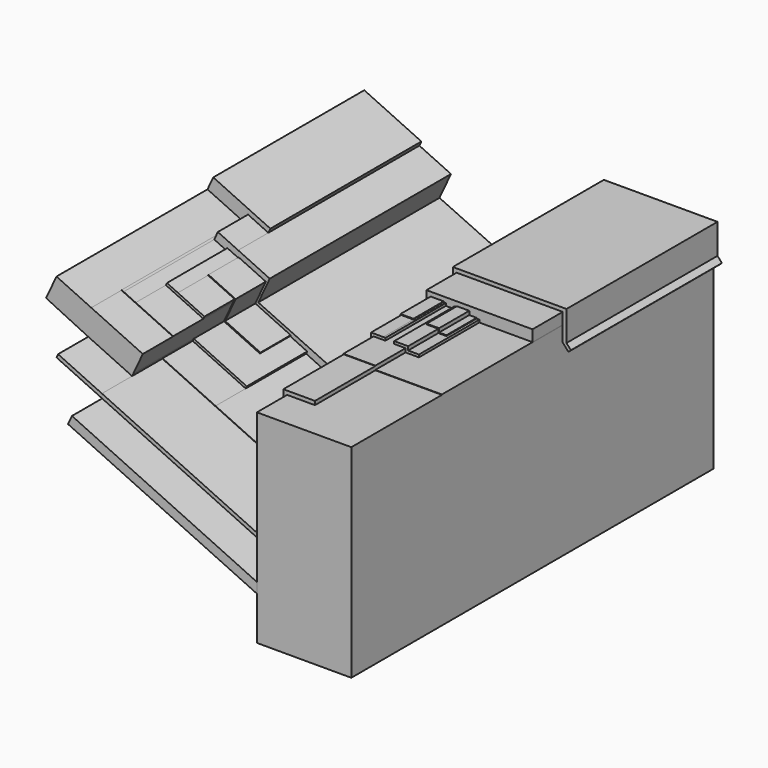
from build123d import *

# Parameters (mm, degrees)
F1_DEPTH  = 120
F2_DEPTH  = 120
F3_DEPTH  = 110
F4_DEPTH  = 100
F5_DEPTH  = 100
F6_DEPTH  = 90
F7_DEPTH  = 90
F8_DEPTH  = 90
F9_DEPTH  = 80
F10_DEPTH = 80
F11_DEPTH = 80
F12_DEPTH = 80
F13_DEPTH = 80
F14_DEPTH = 70
F15_DEPTH = 70
F16_DEPTH = 70
F17_DEPTH = 70
F18_DEPTH = 60
F19_DEPTH = 50
F20_DEPTH = 50


with BuildPart() as f1:
    # F0 (on Front) → F1 (new body)
    with BuildSketch(Plane.XZ):
        Polygon((45.1297726456, 37.9975503451), (37.7532724798, 37.9975503451), (37.7532724798, -1.5682141957), (37.7532724798, -4.3017355894), (37.7532724798, -15.7766969041), (62.7532724798, -15.7766969041), (62.7532724798, 33.9434424275), (62.7532724798, 37.9975503451), align=None)
    extrude(amount=F1_DEPTH)


with BuildPart() as f2:
    # F0 (on Front) → F2 (new body)
    with BuildSketch(Plane.XZ):
        Polygon((37.7532724798, -4.3017355894), (37.7532724798, -1.5682141957), (-11.241981874, 21.2279597303), (-12.2874860827, 18.9808833218), align=None)
    extrude(amount=F2_DEPTH)


with BuildPart() as f3:
    # F0 (on Front) → F3 (new body)
    with BuildSketch(Plane.XZ):
        Polygon((37.7532724798, -1.5682141957), (37.7532724798, 37.9975503451), (45.1297726456, 37.9975503451), (45.1297726456, 38.0975503451), (45.1297726456, 38.9975503451), (36.7532724798, 38.9975503451), (36.7532724798, 9.1857140463), (36.7532724798, 0), (27.1622682206, 4.4624362931), (-11.3030609789, 22.3593192896), (-22.921301212, 27.7649739506), (-23.3431488548, 26.8583072168), (-11.241981874, 21.2279597303), align=None)
    extrude(amount=F3_DEPTH)


with BuildPart() as f4:
    # F0 (on Front) → F4 (new body)
    with BuildSketch(Plane.XZ):
        Polygon((-34.093962769, 33.1498159787), (-22.921301212, 27.7649739506), (-11.3030609789, 22.3593192896), (-11.2608762147, 22.449985963), (-10.978238294, 23.0574526746), (-8.4765384307, 28.4342944867), (-22.1272858391, 34.785620064), (-31.3387730508, 39.0714772835), align=None)
    extrude(amount=F4_DEPTH)


with BuildPart() as f5:
    # F0 (on Front) → F5 (new body)
    with BuildSketch(Plane.XZ):
        Polygon((36.7532724798, 0), (36.7532724798, 9.1857140463), (27.1622682206, 4.4624362931), align=None)
    extrude(amount=F5_DEPTH)


with BuildPart() as f6:
    # F0 (on Front) → F6 (new body)
    with BuildSketch(Plane.XZ):
        Polygon((-22.0851010748, 34.8762867374), (-22.1272858391, 34.785620064), (-8.4765384307, 28.4342944867), (-8.4343536664, 28.5249611601), (-18.3601163214, 33.1431515301), (-21.5557715405, 34.6300039435), align=None)
    extrude(amount=F6_DEPTH)


with BuildPart() as f7:
    # F0 (on Front) → F7 (new body)
    with BuildSketch(Plane.XZ):
        Polygon((36.7532724798, 38.9975503451), (45.1297726456, 38.9975503451), (45.1297726456, 39.0975503451), (42.1224348247, 39.0975503451), (39.793651551, 39.0975503451), (36.6532724798, 39.0975503451), (36.6532724798, 36.1267757076), (36.6532724798, 15.0731514328), (36.6532724798, 9.247935752), (27.1610418439, 4.5733010027), (20.5657351542, 7.641919798), (2.7888639592, 15.9130197845), (-11.2608762147, 22.449985963), (-11.3030609789, 22.3593192896), (27.1622682206, 4.4624362931), (36.7532724798, 9.1857140463), align=None)
    extrude(amount=F7_DEPTH)


with BuildPart() as f8:
    # F0 (on Front) → F8 (new body)
    with BuildSketch(Plane.XZ):
        Polygon((45.1297726456, 38.0975503451), (45.1297726456, 37.9975503451), (62.7532724798, 37.9975503451), (62.7532724798, 38.0975503451), (48.6693568528, 38.0975503451), align=None)
    extrude(amount=F8_DEPTH)


with BuildPart() as f9:
    # F0 (on Front) → F9 (new body)
    with BuildSketch(Plane.XZ):
        Polygon((-18.3601163214, 33.1431515301), (-8.4343536664, 28.5249611601), (-8.1517157457, 29.1324278718), (-15.1795170811, 32.4022747921), (-18.0774784007, 33.7506182417), align=None)
    extrude(amount=F9_DEPTH)


with BuildPart() as f10:
    # F0 (on Front) → F10 (new body)
    with BuildSketch(Plane.XZ):
        Polygon((-10.978238294, 23.0574526746), (-11.2608762147, 22.449985963), (2.7888639592, 15.9130197845), (3.0715018799, 16.5204864961), (-1.4491225171, 18.6238114276), align=None)
    extrude(amount=F10_DEPTH)


with BuildPart() as f11:
    # F0 (on Front) → F11 (new body)
    with BuildSketch(Plane.XZ):
        Polygon((20.987582797, 8.5485865319), (20.5657351542, 7.641919798), (27.1610418439, 4.5733010027), (36.6532724798, 9.247935752), (36.6532724798, 15.0731514328), (35.6532724798, 15.0731514328), (35.6532724798, 13.1126534771), (35.6532724798, 9.8701528088), (27.1487780767, 5.6819480984), (22.5392122095, 7.8266551036), (22.3868255866, 7.8975565001), align=None)
    extrude(amount=F11_DEPTH)


with BuildPart() as f12:
    # F0 (on Front) → F12 (new body)
    with BuildSketch(Plane.XZ):
        Polygon((36.6532724798, 39.0975503451), (39.793651551, 39.0975503451), (39.793651551, 39.7675503451), (39.2196215689, 39.7700648543), (35.9832724798, 39.7842415175), (35.9832724798, 36.6213790533), (35.9832724798, 36.1267757076), (36.6532724798, 36.1267757076), align=None)
    extrude(amount=F12_DEPTH)


with BuildPart() as f13:
    # F0 (on Front) → F13 (new body)
    with BuildSketch(Plane.XZ):
        Polygon((45.1297726456, 38.9975503451), (45.1297726456, 38.0975503451), (48.6693568528, 38.0975503451), (48.6693568528, 38.7675503451), (47.9532927275, 38.7675503451), (45.7997726456, 38.7675503451), (45.7997726456, 39.7675503451), (42.7247062325, 39.7675503451), (42.1224348247, 39.7675503451), (42.1224348247, 39.0975503451), (45.1297726456, 39.0975503451), align=None)
    extrude(amount=F13_DEPTH)


with BuildPart() as f14:
    # F0 (on Front) → F14 (new body)
    with BuildSketch(Plane.XZ):
        Polygon((-8.4765384307, 28.4342944867), (-10.978238294, 23.0574526746), (-1.4491225171, 18.6238114276), (-1.3221520646, 18.8967058894), (-10.6699344948, 23.2459776078), (-7.8860128704, 29.22939169), (-15.0951475526, 32.5836081388), (-15.1795170811, 32.4022747921), (-8.1517157457, 29.1324278718), (-8.4343536664, 28.5249611601), align=None)
    extrude(amount=F14_DEPTH)


with BuildPart() as f15:
    # F0 (on Front) → F15 (new body)
    with BuildSketch(Plane.XZ):
        Polygon((35.6532724798, 9.8701528088), (35.6532724798, 13.1126534771), (35.4532724798, 13.1126534771), (35.4532724798, 9.9945962202), (27.1500502265, 5.9019444203), (22.623581738, 8.0079884503), (22.5392122095, 7.8266551036), (27.1487780767, 5.6819480984), align=None)
    extrude(amount=F15_DEPTH)


with BuildPart() as f16:
    # F0 (on Front) → F16 (new body)
    with BuildSketch(Plane.XZ):
        Polygon((35.9832724798, 39.7842415175), (39.2196215689, 39.7700648543), (39.2196215689, 39.9700648543), (35.7832724798, 39.9700648543), (35.7832724798, 36.6213790533), (35.9832724798, 36.6213790533), align=None)
    extrude(amount=F16_DEPTH)


with BuildPart() as f17:
    # F0 (on Front) → F17 (new body)
    with BuildSketch(Plane.XZ):
        Polygon((45.7997726456, 38.7675503451), (47.9532927275, 38.7675503451), (47.9532927275, 38.9675503451), (45.9997726456, 38.9675503451), (45.9997726456, 39.9675503451), (42.7247062325, 39.9675503451), (42.7247062325, 39.7675503451), (45.7997726456, 39.7675503451), align=None)
    extrude(amount=F17_DEPTH)


with BuildPart() as f18:
    # F0 (on Front) → F18 (new body)
    with BuildSketch(Plane.XZ):
        Polygon((48.6693568528, 38.0975503451), (62.7532724798, 38.0975503451), (62.7532724798, 41.0975503451), (47.1063793285, 41.0975503451), (46.2950781567, 41.0975503451), (34.6532724798, 41.0975503451), (34.6532724798, 33.1212431192), (34.6532724798, 16.1968208849), (33.6532724798, 13.4902799919), (33.6532724798, 11.3371306488), (27.2846735988, 8.1965293972), (23.4195049672, 9.6229607519), (20.8119284671, 9.6229607519), (-9.8889558036, 23.7389743125), (-6.8439622262, 30.2835039038), (-15.2163269439, 34.1789399985), (-20.6001537113, 36.6838897736), (-21.5557715405, 34.6300039435), (-18.3601163214, 33.1431515301), (-18.0774784007, 33.7506182417), (-15.1795170811, 32.4022747921), (-15.0951475526, 32.5836081388), (-7.8860128704, 29.22939169), (-10.6699344948, 23.2459776078), (-1.3221520646, 18.8967058894), (-1.4491225171, 18.6238114276), (3.0715018799, 16.5204864961), (2.7888639592, 15.9130197845), (20.5657351542, 7.641919798), (20.987582797, 8.5485865319), (22.3868255866, 7.8975565001), (22.5392122095, 7.8266551036), (22.623581738, 8.0079884503), (27.1500502265, 5.9019444203), (35.4532724798, 9.9945962202), (35.4532724798, 13.1126534771), (35.6532724798, 13.1126534771), (35.6532724798, 15.0731514328), (36.6532724798, 15.0731514328), (36.6532724798, 36.1267757076), (35.9832724798, 36.1267757076), (35.9832724798, 36.6213790533), (35.7832724798, 36.6213790533), (35.7832724798, 39.9700648543), (39.2196215689, 39.9700648543), (39.2196215689, 39.7700648543), (39.793651551, 39.7675503451), (39.793651551, 39.0975503451), (42.1224348247, 39.0975503451), (42.1224348247, 39.7675503451), (42.7247062325, 39.7675503451), (42.7247062325, 39.9675503451), (45.9997726456, 39.9675503451), (45.9997726456, 38.9675503451), (47.9532927275, 38.9675503451), (47.9532927275, 38.7675503451), (48.6693568528, 38.7675503451), align=None)
    extrude(amount=F18_DEPTH)


with BuildPart() as f19:
    # F0 (on Front) → F19 (new body)
    with BuildSketch(Plane.XZ):
        Polygon((62.7532724798, 38.0975503451), (62.7532724798, 37.9975503451), (62.7532724798, 33.9434424275), (64.2652862209, 32.2634628909), (64.9253694473, 32.85755043), (63.7534983963, 34.1596016824), (63.7534983963, 42.0975503451), (33.6532724798, 42.0975503451), (33.6532724798, 33.7673542435), (32.3305874402, 33.1794772946), (32.7367356742, 32.2656700874), (34.6532724798, 33.1212431192), (34.6532724798, 41.0975503451), (46.2950781567, 41.0975503451), (47.1063793285, 41.0975503451), (62.7532724798, 41.0975503451), align=None)
    extrude(amount=F19_DEPTH)


with BuildPart() as f20:
    # F0 (on Front) → F20 (new body)
    with BuildSketch(Plane.XZ):
        Polygon((-29.8086681311, 42.3600940476), (-31.3387730508, 39.0714772835), (-22.1272858391, 34.785620064), (-22.0851010748, 34.8762867374), (-21.5557715405, 34.6300039435), (-20.6001537113, 36.6838897736), (-15.2163269439, 34.1789399985), (-14.6840246177, 35.323004259), align=None)
    extrude(amount=F20_DEPTH)


solid = Compound([f1.part, f2.part, f3.part, f4.part, f5.part, f6.part, f7.part, f8.part, f9.part, f10.part, f11.part, f12.part, f13.part, f14.part, f15.part, f16.part, f17.part, f18.part, f19.part, f20.part])
